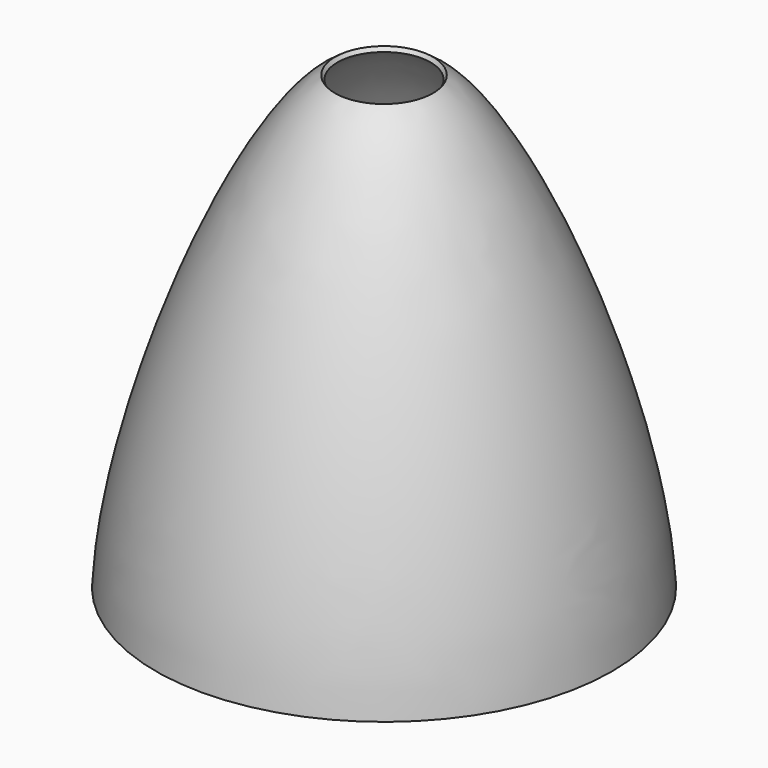
from build123d import *


# Not quite as in the source:
# - the dataset's text gives a spline's control points without its knots; the knots are read off the source's solid


with BuildPart() as f1:
    # F0 (on Front) → F1 (revolve)
    with BuildSketch(Plane.XZ):
        with BuildLine():
            add(Edge.make_bspline(
                [(-127, 0), (-315.2547478676, -118.3398216963), (-588.0008935928, -805.2988312721), (-609.6, -1219.2)],
                knots=[0, 0, 0, 0, 1311.2404051127, 1311.2404051127, 1311.2404051127, 1311.2404051127], degree=3))
            Line((-127, 0), (-133.7589185158, 10.7520738396))
            add(Edge.make_bspline(
                [(-133.7589185158, 10.7520738396), (-140.0815385554, 6.7775779152), (-152.7495279098, -2.2652979505), (-171.8880516902, -18.9159329288), (-191.1948637323, -38.4964920529), (-217.1621757773, -68.3183060606), (-249.9987036601, -112.2086807603), (-289.7034139236, -174.3185013134), (-329.3031723399, -244.7004939723), (-381.3694778118, -347.9847159664), (-443.9169681735, -491.7858839202), (-511.0881247, -678.1471518811), (-566.4810687841, -868.5545883371), (-599.5644066691, -1022.4861292856), (-616.2068474289, -1137.9687978702), (-620.9170609117, -1192.3677004267), (-622.2827457739, -1218.5381609036)],
                knots=[0, 0, 0, 0, 0.03125, 0.0625, 0.09375, 0.125, 0.1875, 0.25, 0.3125, 0.375, 0.5, 0.625, 0.75, 0.875, 0.9375, 1, 1, 1, 1], degree=3))
            Line((-622.2827457739, -1218.5381609036), (-609.6, -1219.2))
        make_face()
    revolve(axis=Axis((0, 0, 31.6490530968), (0, 0, 1)))


solid = f1.part
